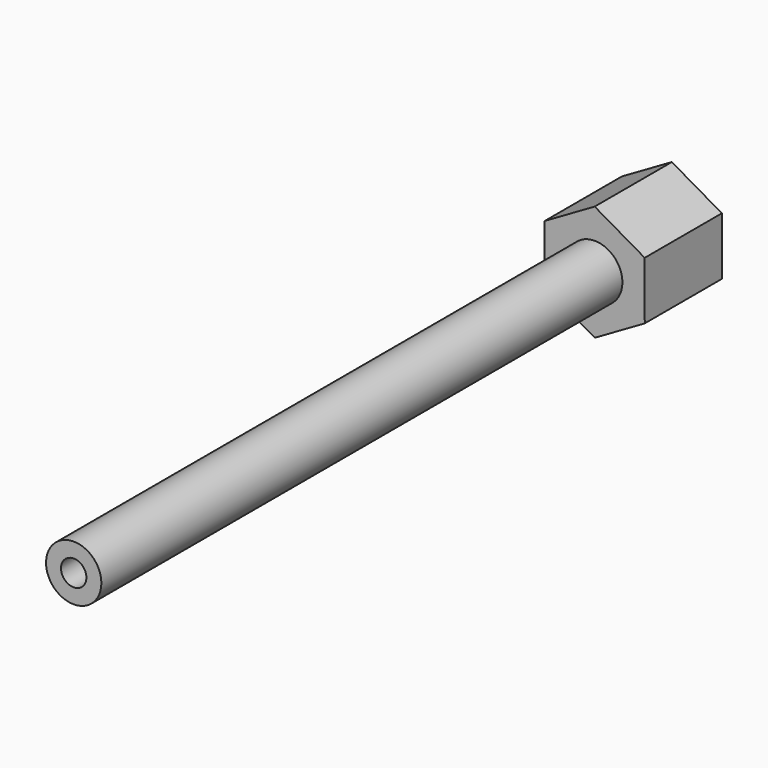
from build123d import *

# Parameters (mm, degrees)
F0_R     = 36.4281701053
F0_R_2   = 16.7456603081
F1_DEPTH = 984.504
F2_DEPTH = 127


# Not quite as in the source:
# - a feature of the source that left no trace in its solid (it failed there, or was rolled back) is left out
# - the program builds the solid bodies; features that only make, move or delete a surface that nothing else refers to are left out


with BuildPart() as f1:
    # F0 (on Front) → F1 (new body)
    with BuildSketch(Plane.XZ):
        Circle(F0_R)
        Circle(F0_R_2, mode=Mode.SUBTRACT)
    extrude(amount=F1_DEPTH)

    # F0 (on Front) → F2 (join)
    with BuildSketch(Plane.XZ):
        Polygon((0.0695483181, -76.0122935755), (65.8633513954, -37.9459161775), (65.7938030773, 38.0663773981), (-0.0695483181, 76.0122935755), (-65.8633513954, 37.9459161775), (-65.7938030773, -38.0663773981), align=None)
        Circle(F0_R, mode=Mode.SUBTRACT)
    extrude(amount=F2_DEPTH)


solid = f1.part
